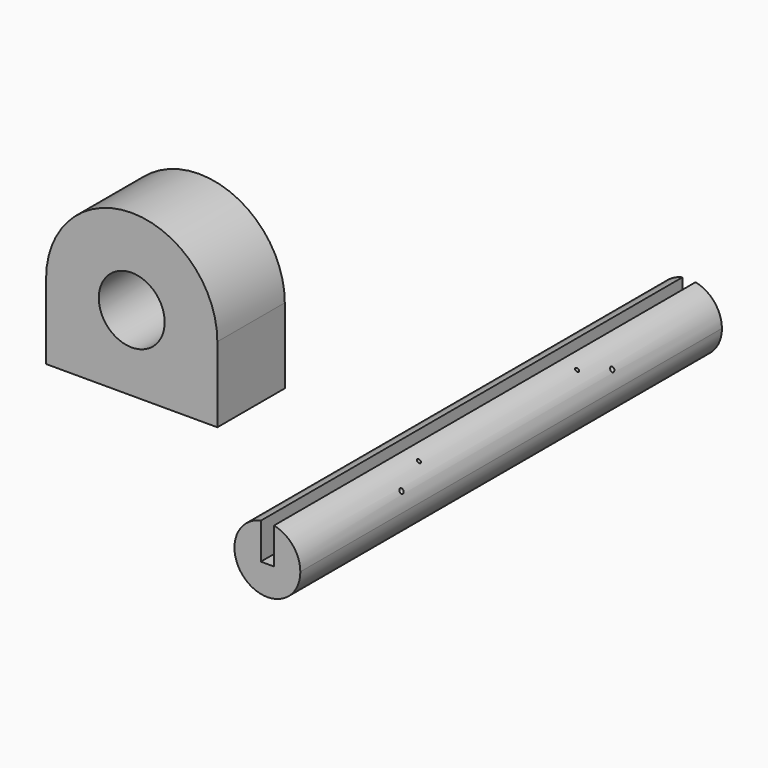
from build123d import *

# Parameters (mm, degrees)
F0_R           = 25
F1_DEPTH       = 64
F3_DEPTH       = 200
F6_D           = 3.3
F6_DEPTH       = 20.001
F6_ON_F5_D     = 3.3
F6_ON_F5_DEPTH = 20.001
F8_D           = 2.5
F8_DEPTH       = 25
F8_TIP         = 0.7510757738
F10_D          = 14
F10_DEPTH      = 35
F10_TIP        = 4.2060243332


# Not quite as in the source:
# - a feature names something its author has since deleted; it is built from what else it names


with BuildPart() as f1:
    # F0 (on Front) → F1 (new body)
    with BuildSketch(Plane.XZ):
        with BuildLine():
            Line((65, -57.2), (65, 0))
            ThreePointArc((65, 0), (0, 65), (-65, 0))
            Line((-65, 0), (-65, -57.2))
            Line((-65, -57.2), (0, -57.2))
            Line((0, -57.2), (65, -57.2))
        make_face()
        Circle(F0_R, mode=Mode.SUBTRACT)
    extrude(amount=-F1_DEPTH)

    # F10
    with Locations(Plane(origin=(0, 0, -57.2), x_dir=(1, 0, 0), z_dir=(0, 0, -1))):
        with Locations((-47, -32), (47, -32)):
            Hole(F10_D / 2, depth=F10_DEPTH)
            with Locations((0, 0, -(F10_DEPTH + F10_TIP / 2))):  # 118° drill point
                Cone(0, F10_D / 2, F10_TIP, mode=Mode.SUBTRACT)


with BuildPart() as f3:
    # F2 (on Front) → F3 (new body, symmetric)
    with BuildSketch(Plane.XZ):
        with BuildLine():
            ThreePointArc((237.9897642136, 0), (263.0397643136, -24.9999499997), (287.9895642128, 0.1))
            ThreePointArc((287.9895642128, 0.1), (282.3230193747, 15.8500865888), (267.9897642136, 24.4948974278))
            Line((267.9897642136, 24.4948974278), (267.9897642136, -2.9))
            Line((267.9897642136, -2.9), (257.9897642136, -2.9))
            Line((257.9897642136, -2.9), (257.9897642136, 24.4948974278))
            ThreePointArc((257.9897642136, 24.4948974278), (243.6248474825, 15.8113883008), (237.9897642136, 0))
        make_face()
    extrude(amount=F3_DEPTH, both=True)

    # F6 (through all, one way)
    with BuildSketch(Plane.YZ.offset(257.9897642136)):
        with Locations((100, 12.2474487139), (-100, 12.2474487139)):
            Circle(F6_D / 2)
    extrude(amount=-F6_DEPTH, mode=Mode.SUBTRACT)

    # F6 on F5 (through all, one way)
    with BuildSketch(Plane(origin=(267.9897642136, 0, 0), x_dir=(0, -1, 0), z_dir=(-1, 0, 0))):
        with Locations((-100, 12.2474487139), (100, 12.2474487139)):
            Circle(F6_ON_F5_D / 2)
    extrude(amount=-F6_ON_F5_DEPTH, mode=Mode.SUBTRACT)

    # F8 (one way)
    with BuildSketch(Plane(origin=(0, 0, -2.9), x_dir=(1, 0, 0), z_dir=(0, 0, -1))):
        with Locations((247.9897642136, 75), (277.9897642136, 75), (277.9897642136, -75), (247.9897642136, -75)):
            Circle(F8_D / 2)
    extrude(amount=-F8_DEPTH, mode=Mode.SUBTRACT)
    with Locations(Plane(origin=(0, 0, -2.9), x_dir=(1, 0, 0), z_dir=(0, 0, -1))):
        with Locations((247.9897642136, 75), (277.9897642136, 75), (277.9897642136, -75), (247.9897642136, -75)):
            with Locations((0, 0, -(F8_DEPTH + F8_TIP / 2))):  # 118° drill point
                Cone(0, F8_D / 2, F8_TIP, mode=Mode.SUBTRACT)


solid = Compound([f1.part, f3.part])
